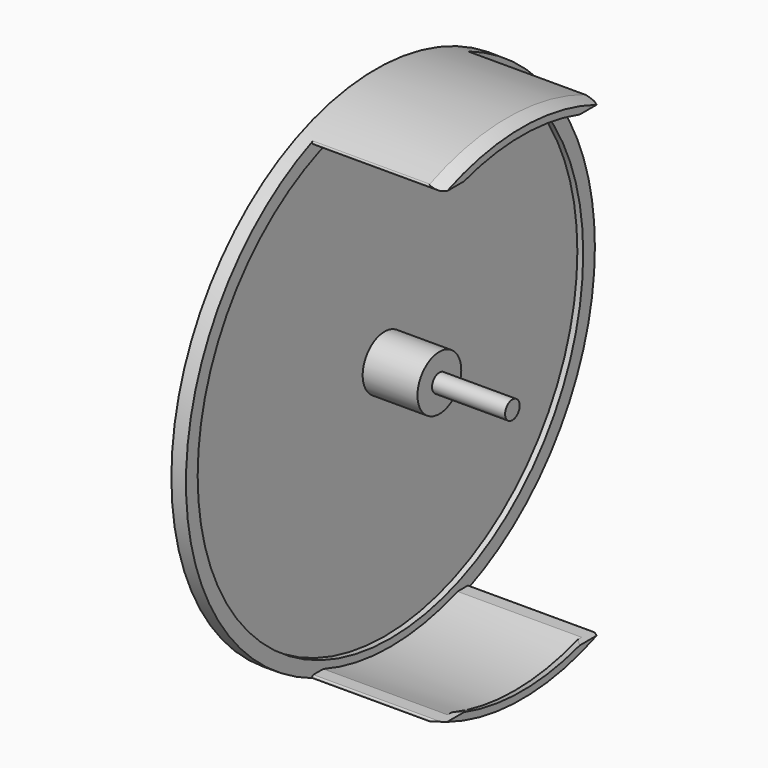
from build123d import *

# Parameters (mm, degrees)
F0_R       = 44.45
F1_DEPTH   = 25.4
F2_R       = 43.18
F3_DEPTH   = 22.86
F4_R       = 44.45
F4_R_2     = 42.545
F5_DEPTH   = 1.27
F6_W       = 25.4
F6_H       = 81.28
F7_DEPTH   = 63.5
F8_SIZE2   = 0.340285
F8_SIZE    = 1.26999
F8_2_SIZE2 = 0.340285
F8_2_SIZE  = 1.26999
F9_SIZE2   = 0.6805909488
F9_SIZE    = 2.54
F10_R      = 0.254
F11_R      = 41.91
F12_DEPTH  = 1.016
F13_R      = 4.7625
F14_DEPTH  = 9.525
F15_R      = 1.5875
F16_DEPTH  = 12.7


# Not quite as in the source:
# - a fillet or chamfer is up to 0.001 mm smaller than in the source, because OpenCascade refuses the exact size


with BuildPart() as f1:
    # F0 (on Right) → F1 (new body)
    with BuildSketch(Plane.YZ):
        Circle(F0_R)
    extrude(amount=F1_DEPTH)

    # F2 (on face) → F3 (cut)
    with BuildSketch(Plane.YZ.offset(25.4)):
        Circle(F2_R)
    extrude(amount=-F3_DEPTH, mode=Mode.SUBTRACT)

    # F4 (on face) → F5 (join)
    with BuildSketch(Plane.YZ.offset(25.4)):
        Circle(F4_R)
        Circle(F4_R_2, mode=Mode.SUBTRACT)
    extrude(amount=-F5_DEPTH)

    # F6 (on Front) → F7 (cut, symmetric)
    with BuildSketch(Plane.XZ):
        with Locations((15.24, 0)):
            Rectangle(F6_W, F6_H)
    extrude(amount=F7_DEPTH, both=True, mode=Mode.SUBTRACT)

    # F8 (size 1.27 and 0.3402954744 in the source; OpenCascade refuses exactly that, so slightly less here)
    f8_edges = [f1.edges().sort_by_distance(p)[0] for p in [
        (24.13, 0, -42.545),
    ]]
    f8_side = f1.faces().sort_by_distance((24.765, 0, -42.545))[0]
    chamfer(f8_edges, length=F8_SIZE, length2=F8_SIZE2, reference=f8_side)

    # F8#2 (size 1.27 and 0.3402954744 in the source; OpenCascade refuses exactly that, so slightly less here)
    f8_2_edges = [f1.edges().sort_by_distance(p)[0] for p in [
        (24.13, 0, 42.545),
    ]]
    f8_2_side = f1.faces().sort_by_distance((24.765, 0, 42.545))[0]
    chamfer(f8_2_edges, length=F8_2_SIZE, length2=F8_2_SIZE2, reference=f8_2_side)

    # F9
    f9_edges = [f1.edges().sort_by_distance(p)[0] for p in [
        (25.4, 0, -44.45),
        (25.4, 0, 44.45),
    ]]
    f9_side = f1.faces().sort_by_distance((1.257363, 37.256816, -24.243188))[0]
    chamfer(f9_edges, length=F9_SIZE, length2=F9_SIZE2, reference=f9_side)

    # F10
    f10_edges = [f1.edges().sort_by_distance(p)[0] for p in [
        (12.7, 18.005358, -40.64),
        (12.7, -18.005358, -40.64),
        (12.7, -18.005358, 40.64),
        (12.7, 18.005358, 40.64),
    ]]
    fillet(f10_edges, radius=F10_R)

    # F11 (on face) → F12 (cut)
    with BuildSketch(Plane.YZ.offset(2.54)):
        Circle(F11_R)
    extrude(amount=-F12_DEPTH, mode=Mode.SUBTRACT)

    # F13 (on face) → F14 (join)
    with BuildSketch(Plane.YZ.offset(1.524)):
        Circle(F13_R)
    extrude(amount=F14_DEPTH)

    # F15 (on face) → F16 (join)
    with BuildSketch(Plane.YZ.offset(11.049)):
        Circle(F15_R)
    extrude(amount=F16_DEPTH)


solid = f1.part
